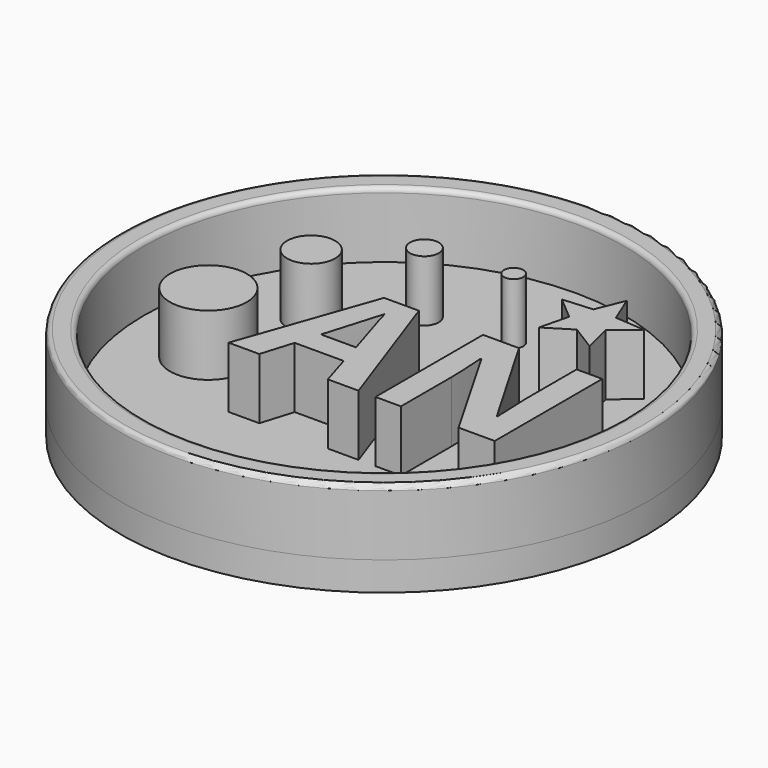
from build123d import *

# Parameters (mm, degrees)
F0_R         = 27.5
F0_R_2       = 25
F0_R_3       = 4
F0_R_4       = 2.5
F0_TEXT_SIZE = 19.621524474
F0_R_5       = 1
F0_R_6       = 1.5
F1_DEPTH     = 6.35
F2_R         = 27.5
F3_DEPTH     = 3
F4_DEPTH     = 0.5
F5_R         = 0.5


# Not quite as in the source:
# - Text() gives the source's letters only with a copy of the font that has no kerning and outlines rounded to 1/6400 em; it was checked with that copy


with BuildPart() as f1:
    # F0 (on Top) → F1 (new body)
    with BuildSketch(Plane.XY):
        Circle(F0_R)
        Circle(F0_R_2, mode=Mode.SUBTRACT)
        with Locations((-16.3095064303, -2.5)):
            Circle(F0_R_3)
        with Locations((-14, 8)):
            Circle(F0_R_4)
        with Locations((-9, -9)):
            Text('AN', F0_TEXT_SIZE, font='Open Sans', font_style=FontStyle.BOLD, text_align=(TextAlign.LEFT, TextAlign.BOTTOM))
        Polygon((12.8607498028, 14.1180339887), (11.6851792982, 17), (10.5096087936, 14.1180339887), (7.4054249749, 13.8905764747), (9.7830662656, 11.8819660113), (9.0401456629, 8.8594235253), (11.6851792982, 10.5), (14.3302129335, 8.8594235253), (13.5872923308, 11.8819660113), (15.9649336216, 13.8905764747), align=None)
        with Locations((1.5, 15)):
            Circle(F0_R_5)
        with Locations((-7, 14)):
            Circle(F0_R_6)
    extrude(amount=F1_DEPTH)

    # F4 (add): a face of the model
    f4_faces = [f1.faces().sort_by_distance(p)[0] for p in [
        (-26.7221825407, 0, 6.35),
    ]]
    extrude(f4_faces, amount=F4_DEPTH)

    # F5
    f5_edges = [f1.edges().sort_by_distance(p)[0] for p in [
        (-27.5, 0, 6.85),
        (-25, 0, 6.85),
    ]]
    fillet(f5_edges, radius=F5_R)


with BuildPart() as f3:
    # F2 (on Top) → F3 (new body)
    with BuildSketch(Plane.XY):
        Circle(F2_R)
    extrude(amount=-F3_DEPTH)


solid = Compound([f1.part, f3.part])
